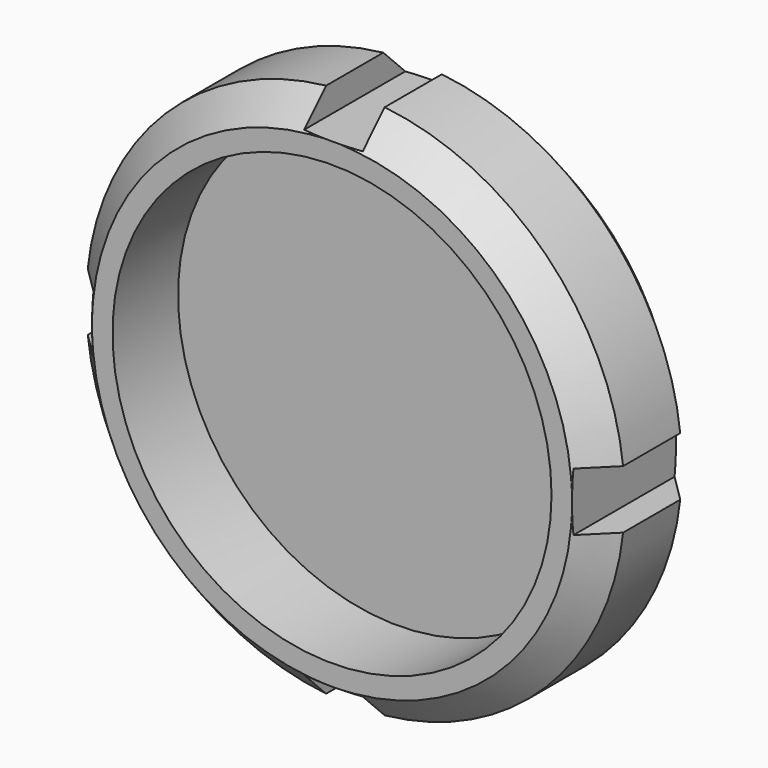
from build123d import *

# Parameters (mm, degrees)
F0_R             = 46
F1_DEPTH         = 22.5
F2_T             = -8.5
F3_R             = 55.4976575172
F3_R_2           = 39
F4_DEPTH         = 0.3
F5_R             = 5
F6_DEPTH         = 6
F7_R             = 7.5
F7_R_2           = 5
F8_DEPTH         = 5
F9_SIZE2         = 5
F9_SIZE          = 5
F10_W            = 11.5703346615
F10_H            = 10
F11_DEPTH        = 22.501
F11_COPIES_COUNT = 4


# Not quite as in the source:
# - a pattern or mirror of a feature is missing from the dataset's text; its kind, count and spacing are read off the source's solid


with BuildPart() as f1:
    # F0 (on Front) → F1 (new body)
    with BuildSketch(Plane.XZ):
        Circle(F0_R)
    extrude(amount=F1_DEPTH)

    # F2
    f2_openings = [f1.faces().sort_by_distance(p)[0] for p in [
        (0, -22.5, 0),
    ]]
    offset(amount=F2_T, openings=f2_openings)

    # F3 (on Front) → F4 (cut)
    with BuildSketch(Plane.XZ):
        Circle(F3_R)
        Circle(F3_R_2, mode=Mode.SUBTRACT)
    extrude(amount=F4_DEPTH, mode=Mode.SUBTRACT)

    # F5 (on Front) → F6 (join)
    with BuildSketch(Plane.XZ):
        Circle(F5_R)
    extrude(amount=-F6_DEPTH)

    # F7 (on face) → F8 (join)
    with BuildSketch(Plane(origin=(0, 6, 0), x_dir=(-1, 0, 0), z_dir=(0, 1, 0))):
        Circle(F7_R)
        Circle(F7_R_2, mode=Mode.SUBTRACT)
        Circle(F7_R_2)
    extrude(amount=F8_DEPTH)

    # F9
    f9_edges = [f1.edges().sort_by_distance(p)[0] for p in [
        (-46, -0.3, 0),
        (-46, -22.5, 0),
    ]]
    chamfer(f9_edges, length=F9_SIZE, length2=F9_SIZE2)

    # F10 (on Front) → F11 (cut, through all)
    with BuildSketch(Plane.XZ):
        with Locations((46.7851673308, 0)):
            Rectangle(F10_W, F10_H)
    f11 = extrude(amount=F11_DEPTH, mode=Mode.SUBTRACT)

    # F11_copies: F11 ×4 about axis
    f11_copies_axis = Axis((0, 0, 0), (0, 1, 0))
    for i in range(1, F11_COPIES_COUNT):
        add(f11.rotate(f11_copies_axis, i * 360 / F11_COPIES_COUNT), mode=Mode.SUBTRACT)


solid = f1.part
